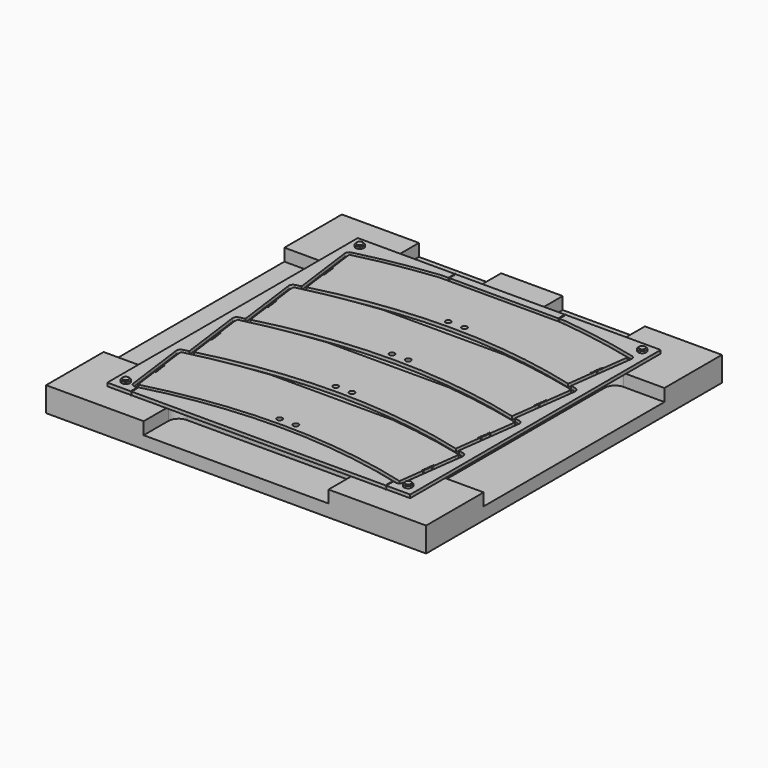
from build123d import *

# Parameters (mm, degrees)
F0_W     = 185
F0_H     = 180
F1_DEPTH = 12
F3_DEPTH = 6
F4_R     = 2.0005
F4_R_2   = 0.3015
F5_DEPTH = 1.6
F4_R_3   = 1.3005
F6_R     = 1.95
F7_DEPTH = 3
F8_SIZE  = 0.5


# Not quite as in the source:
# - ends of sketch curves that miss each other by under 0.0002 mm in the source are joined


with BuildPart() as f1:
    # F0 (on Top) → F1 (new body)
    with BuildSketch(Plane.XY):
        Rectangle(F0_W, F0_H)
    extrude(amount=F1_DEPTH)

    # F2 (on face) → F3 (cut)
    with BuildSketch(Plane.XY.offset(12)):
        with BuildLine():
            Line((117.5, -55), (117.5, 55))
            Line((117.5, 55), (72.5, 55))
            ThreePointArc((72.5, 55), (68.9644660941, 53.5355339059), (67.5, 50))
            Line((67.5, 50), (67.5, -50))
            ThreePointArc((67.5, -50), (68.9644660941, -53.5355339059), (72.5, -55))
            Line((72.5, -55), (117.5, -55))
        make_face()
        with BuildLine():
            ThreePointArc((45, -75), (43.5355339059, -71.4644660941), (40, -70))
            Line((40, -70), (-40, -70))
            ThreePointArc((-40, -70), (-43.5355339059, -71.4644660941), (-45, -75))
            Line((-45, -75), (-45, -110))
            Line((-45, -110), (45, -110))
            Line((45, -110), (45, -75))
        make_face()
        with BuildLine():
            Line((55, 77), (55, 108))
            Line((55, 108), (15, 108))
            Line((15, 108), (15, 77))
            ThreePointArc((15, 77), (16.4644660941, 73.4644660941), (20, 72))
            Line((20, 72), (50, 72))
            ThreePointArc((50, 72), (53.5355339059, 73.4644660941), (55, 77))
        make_face()
        with BuildLine():
            Line((-15, 108), (-55, 108))
            Line((-55, 108), (-55, 77))
            ThreePointArc((-55, 77), (-53.5355339059, 73.4644660941), (-50, 72))
            Line((-50, 72), (-20, 72))
            ThreePointArc((-20, 72), (-16.4644660941, 73.4644660941), (-15, 77))
            Line((-15, 77), (-15, 108))
        make_face()
        with BuildLine():
            ThreePointArc((-67.5, 50), (-68.9644660941, 53.5355339059), (-72.5, 55))
            Line((-72.5, 55), (-117.5, 55))
            Line((-117.5, 55), (-117.5, -55))
            Line((-117.5, -55), (-72.5, -55))
            ThreePointArc((-72.5, -55), (-68.9644660941, -53.5355339059), (-67.5, -50))
            Line((-67.5, -50), (-67.5, 50))
        make_face()
    extrude(amount=-F3_DEPTH, mode=Mode.SUBTRACT)

    # F6 (on face) → F7 (join)
    with BuildSketch(Plane.XY.offset(12)):
        with Locations((68.726, 71.2005)):
            Circle(F6_R)
        with Locations((-68.726, 71.2005)):
            Circle(F6_R)
        with Locations((68.726, -71.2005)):
            Circle(F6_R)
        with Locations((-68.726, -71.2005)):
            Circle(F6_R)
    extrude(amount=F7_DEPTH)

    # F8
    f8_edges = [f1.edges().sort_by_distance(p)[0] for p in [
        (-70.676, -71.2005, 15),
        (66.776, -71.2005, 15),
        (66.776, 71.2005, 15),
        (-70.676, 71.2005, 15),
    ]]
    chamfer(f8_edges, length=F8_SIZE)


with BuildPart() as f5:
    # F4 (on face) → F5 (new body)
    with BuildSketch(Plane.XY.offset(12)):
        with BuildLine():
            Line((-62.4545, -76.2005), (-61.8515, -76.2005))
            ThreePointArc((-61.8515, -76.2005), (-62.153, -75.899), (-62.4545, -76.2005))
        make_face()
        with BuildLine():
            ThreePointArc((-62.4545, -76.2005), (-62.153, -75.899), (-61.8515, -76.2005))
            Line((-61.8515, -76.2005), (61.5455, -76.2005))
            ThreePointArc((61.5455, -76.2005), (61.847, -75.899), (62.1485, -76.2005))
            Line((62.1485, -76.2005), (73.726, -76.2005))
            Line((73.726, -76.2005), (73.726, 76.2005))
            Line((73.726, 76.2005), (27.6285, 76.2005))
            ThreePointArc((27.6285, 76.2005), (27.327, 75.899), (27.0255, 76.2005))
            Line((27.0255, 76.2005), (-25.9215, 76.2005))
            ThreePointArc((-25.9215, 76.2005), (-26.223, 75.899), (-26.5245, 76.2005))
            Line((-26.5245, 76.2005), (-73.726, 76.2005))
            Line((-73.726, 76.2005), (-73.726, -76.2005))
            Line((-73.726, -76.2005), (-62.4545, -76.2005))
        make_face()
        with Locations((-68.726, -71.2005)):
            Circle(F4_R, mode=Mode.SUBTRACT)
        with Locations((-62.153, -75.2505)):
            Circle(F4_R_2, mode=Mode.SUBTRACT)
        with Locations((-62.153, -74.3005)):
            Circle(F4_R_2, mode=Mode.SUBTRACT)
        with Locations((-62.153, -73.3505)):
            Circle(F4_R_2, mode=Mode.SUBTRACT)
        with Locations((-62.153, -72.4005)):
            Circle(F4_R_2, mode=Mode.SUBTRACT)
        with Locations((61.847, -75.2505)):
            Circle(F4_R_2, mode=Mode.SUBTRACT)
        with Locations((61.847, -74.3005)):
            Circle(F4_R_2, mode=Mode.SUBTRACT)
        with Locations((61.847, -73.3505)):
            Circle(F4_R_2, mode=Mode.SUBTRACT)
        with Locations((61.847, -72.4005)):
            Circle(F4_R_2, mode=Mode.SUBTRACT)
        with Locations((68.726, -71.2005)):
            Circle(F4_R, mode=Mode.SUBTRACT)
        with BuildLine():
            Line((-65.62, -70.4485), (-67.2449358727, -58.1074915558))
            Line((-67.2449358727, -58.1074915558), (-69.709, -39.3935))
            ThreePointArc((-69.709, -39.3935), (-69.3772702277, -38.004016098), (-68.2030000316, -37.1904998711))
            Line((-68.2030000316, -37.1904998711), (-66.882, -36.8665))
            Line((-66.882, -36.8665), (-65.559, -36.5485))
            Line((-65.559, -36.5485), (-65.595, -36.3995))
            Line((-65.595, -36.3995), (-65.62, -36.2485))
            Line((-65.62, -36.2485), (-67.2450652985, -23.9065085973))
            Line((-67.2450652985, -23.9065085973), (-69.709, -5.1935))
            ThreePointArc((-69.709, -5.1935), (-69.3770638062, -3.8037858875), (-68.2029999873, -2.9895000517))
            Line((-68.2029999873, -2.9895000517), (-66.882, -2.6655))
            Line((-66.882, -2.6655), (-65.559, -2.3485))
            Line((-65.559, -2.3485), (-65.595, -2.1995))
            Line((-65.595, -2.1995), (-65.62, -2.0475))
            Line((-65.62, -2.0475), (-67.2449358727, 10.2935084442))
            Line((-67.2449358727, 10.2935084442), (-69.709, 29.0075))
            ThreePointArc((-69.709, 29.0075), (-69.3767664611, 30.3966415962), (-68.2030001005, 31.2105004081))
            Line((-68.2030001005, 31.2105004081), (-66.882, 31.5345))
            Line((-66.882, 31.5345), (-65.559, 31.8525))
            Line((-65.559, 31.8525), (-65.595, 32.0015))
            Line((-65.595, 32.0015), (-65.62, 32.1525))
            Line((-65.62, 32.1525), (-67.2449358727, 44.4935084442))
            Line((-67.2449358727, 44.4935084442), (-69.709, 63.2075))
            ThreePointArc((-69.709, 63.2075), (-69.3772702277, 64.596983902), (-68.2030000316, 65.4105001289))
            ThreePointArc((-68.2030000316, 65.4105001289), (-49.0501556944, 69.4631942467), (-29.6639999694, 72.1894997101))
            Line((-29.6639999694, 72.1894997101), (-29.557, 72.1985))
            Line((-29.557, 72.1985), (-29.449, 72.2015))
            Line((-29.449, 72.2015), (-26.4494533888, 72.201449472))
            ThreePointArc((-26.4494533888, 72.201449472), (-26.3293638879, 72.6826151775), (-25.9215, 72.4005))
            ThreePointArc((-25.9215, 72.4005), (-25.9408866143, 72.2941313599), (-25.9965533175, 72.2014418428))
            Line((-25.9965533175, 72.2014418428), (27.1013427235, 72.2005473967))
            ThreePointArc((27.1013427235, 72.2005473967), (27.2200734338, 72.6824023934), (27.6285, 72.4005))
            ThreePointArc((27.6285, 72.4005), (27.6089005922, 72.2935686851), (27.5526505399, 72.2005397943))
            Line((27.5526505399, 72.2005397943), (29.915, 72.2005))
            Line((29.915, 72.2005), (29.924, 72.2005))
            Line((29.924, 72.2005), (30.031, 72.1975))
            Line((30.031, 72.1975), (30.137, 72.1885))
            ThreePointArc((30.137, 72.1885), (49.2837916508, 69.5048541336), (68.2040000196, 65.5265000796))
            ThreePointArc((68.2040000196, 65.5265000796), (69.3770080847, 64.7122741999), (69.7089998684, 63.3235000172))
            Line((69.7089998684, 63.3235000172), (68.0082998947, 50.4077430393))
            Line((68.0082998947, 50.4077430393), (67.2342399079, 44.5292400436))
            Line((67.2342399079, 44.5292400436), (65.619, 32.2625))
            Line((65.619, 32.2625), (65.594, 32.1115))
            Line((65.594, 32.1115), (65.557, 31.9635))
            Line((65.557, 31.9635), (66.881, 31.6475))
            Line((66.881, 31.6475), (68.204, 31.3255))
            ThreePointArc((68.204, 31.3255), (69.3774420415, 30.5115704613), (69.7090000669, 29.1224999912))
            Line((69.7090000669, 29.1224999912), (68.0089998907, 16.212059072))
            Line((68.0089998907, 16.212059072), (67.2342480853, 10.3283021459))
            Line((67.2342480853, 10.3283021459), (65.619, -1.9385))
            Line((65.619, -1.9385), (65.594, -2.0885))
            Line((65.594, -2.0885), (65.557, -2.2365))
            Line((65.557, -2.2365), (66.881, -2.5525))
            Line((66.881, -2.5525), (68.204, -2.8745))
            ThreePointArc((68.204, -2.8745), (69.3770080847, -3.6887258001), (69.7089998684, -5.0774999828))
            Line((69.7089998684, -5.0774999828), (68.0089998907, -17.987940928))
            Line((68.0089998907, -17.987940928), (67.2342399079, -23.8717599564))
            Line((67.2342399079, -23.8717599564), (65.619, -36.1385))
            Line((65.619, -36.1385), (65.594, -36.2895))
            Line((65.594, -36.2895), (65.557, -36.4365))
            Line((65.557, -36.4365), (66.881, -36.7525))
            Line((66.881, -36.7525), (68.204, -37.0745))
            ThreePointArc((68.204, -37.0745), (69.3770080847, -37.8887258001), (69.7089998684, -39.2774999828))
            Line((69.7089998684, -39.2774999828), (69.709, -39.2785))
            Line((69.709, -39.2785), (68.0098089454, -52.1827966615))
            Line((68.0098089454, -52.1827966615), (67.233899191, -58.0753474888))
            Line((67.233899191, -58.0753474888), (65.619, -70.3395))
            ThreePointArc((65.619, -70.3395), (64.749919219, -71.7392145375), (63.1250000615, -72.0114997676))
            ThreePointArc((63.1250000615, -72.0114997676), (-0.0064015619, -63.8958856781), (-63.1220000549, -72.1334997925))
            Line((-63.1220000549, -72.1334997925), (-63.124, -72.1335))
            ThreePointArc((-63.124, -72.1335), (-64.7548109583, -71.858060865), (-65.62, -70.4485))
        make_face(mode=Mode.SUBTRACT)
        with Locations((-68.726, 71.2005)):
            Circle(F4_R, mode=Mode.SUBTRACT)
        with Locations((-26.223, 73.3505)):
            Circle(F4_R_2, mode=Mode.SUBTRACT)
        with Locations((-26.223, 74.3005)):
            Circle(F4_R_2, mode=Mode.SUBTRACT)
        with Locations((-26.223, 75.2505)):
            Circle(F4_R_2, mode=Mode.SUBTRACT)
        with Locations((27.327, 73.3505)):
            Circle(F4_R_2, mode=Mode.SUBTRACT)
        with Locations((27.327, 74.3005)):
            Circle(F4_R_2, mode=Mode.SUBTRACT)
        with Locations((27.327, 75.2505)):
            Circle(F4_R_2, mode=Mode.SUBTRACT)
        with Locations((68.726, 71.2005)):
            Circle(F4_R, mode=Mode.SUBTRACT)
        with BuildLine():
            ThreePointArc((-62.4545, -76.2005), (-62.153, -76.502), (-61.8515, -76.2005))
            Line((-61.8515, -76.2005), (-62.4545, -76.2005))
        make_face()
        with BuildLine():
            Line((62.1485, -76.2005), (61.5455, -76.2005))
            ThreePointArc((61.5455, -76.2005), (61.847, -76.502), (62.1485, -76.2005))
        make_face()
        with BuildLine():
            ThreePointArc((62.1485, -76.2005), (61.847, -75.899), (61.5455, -76.2005))
            Line((61.5455, -76.2005), (62.1485, -76.2005))
        make_face()
        with BuildLine():
            Line((-25.9215, 76.2005), (-26.5245, 76.2005))
            ThreePointArc((-26.5245, 76.2005), (-26.223, 75.899), (-25.9215, 76.2005))
        make_face()
        with BuildLine():
            ThreePointArc((-25.9215, 76.2005), (-26.223, 76.502), (-26.5245, 76.2005))
            Line((-26.5245, 76.2005), (-25.9215, 76.2005))
        make_face()
        with BuildLine():
            Line((27.0255, 76.2005), (27.6285, 76.2005))
            ThreePointArc((27.6285, 76.2005), (27.327, 76.502), (27.0255, 76.2005))
        make_face()
        with BuildLine():
            ThreePointArc((27.0255, 76.2005), (27.327, 75.899), (27.6285, 76.2005))
            Line((27.6285, 76.2005), (27.0255, 76.2005))
        make_face()
    extrude(amount=F5_DEPTH)


with BuildPart() as f5b:
    # F4 (on face) → F5, piece 2 (new body)
    with BuildSketch(Plane.XY.offset(12)):
        with BuildLine():
            Line((-65.2784456317, 44.8756615856), (-65.2664345686, 44.784424493))
            Line((-65.2664345686, 44.784424493), (-63.636, 32.3995))
            ThreePointArc((-63.636, 32.3995), (-0.007966778, 40.7044773709), (63.6359999804, 32.5224999254))
            Line((63.6359999804, 32.5224999254), (63.637, 32.5225))
            Line((63.637, 32.5225), (65.247008228, 44.7524989168))
            Line((65.247008228, 44.7524989168), (65.2625989091, 44.8709293753))
            ThreePointArc((65.2625989091, 44.8709293753), (64.669481786, 44.9740121639), (65.2705, 44.9395))
            ThreePointArc((65.2705, 44.9395), (65.2704605754, 44.934624399), (65.2703423119, 44.9297500732))
            Line((65.2703423119, 44.9297500732), (65.3866191433, 45.8130160697))
            ThreePointArc((65.3866191433, 45.8130160697), (64.793476694, 45.9159679438), (65.3945, 45.8815))
            ThreePointArc((65.3945, 45.8815), (65.3944598523, 45.8765798927), (65.3943394199, 45.8716610957))
            Line((65.3943394199, 45.8716610957), (65.5106394125, 46.7551030307))
            ThreePointArc((65.5106394125, 46.7551030307), (64.9174715933, 46.8579235902), (65.5185, 46.8235))
            ThreePointArc((65.5185, 46.8235), (65.5184591204, 46.8185352527), (65.5183364928, 46.8135718517))
            Line((65.5183364928, 46.8135718517), (65.6346597172, 47.6971902605))
            ThreePointArc((65.6346597172, 47.6971902605), (65.0414664837, 47.7998791017), (65.6425, 47.7655))
            ThreePointArc((65.6425, 47.7655), (65.6424583797, 47.7604904779), (65.6423335303, 47.7554823389))
            Line((65.6423335303, 47.7554823389), (65.7586800576, 48.6392777617))
            ThreePointArc((65.7586800576, 48.6392777617), (65.1654613653, 48.7418344772), (65.7665, 48.7075))
            ThreePointArc((65.7665, 48.7075), (65.76645763, 48.7024455671), (65.7663305321, 48.6973925547))
            Line((65.7663305321, 48.6973925547), (65.882700434, 49.5813655368))
            ThreePointArc((65.882700434, 49.5813655368), (65.2894562379, 49.6837897153), (65.8905, 49.6495))
            ThreePointArc((65.8905, 49.6495), (65.8904568714, 49.6444005189), (65.8903274978, 49.6393024967))
            Line((65.8903274978, 49.6393024967), (66.0067208468, 50.5234535882))
            ThreePointArc((66.0067208468, 50.5234535882), (65.4134511014, 50.6257448149), (66.0145, 50.5915))
            ThreePointArc((66.0145, 50.5915), (66.0144561036, 50.5863553321), (66.0143244271, 50.5812121623))
            Line((66.0143244271, 50.5812121623), (66.0300275006, 50.7004963797))
            Line((66.0300275006, 50.7004963797), (67.726, 63.5835))
            ThreePointArc((67.726, 63.5835), (48.9375198691, 67.5344075087), (29.9239999395, 70.1994994278))
            Line((29.9239999395, 70.1994994278), (-29.449, 70.2005))
            ThreePointArc((-29.449, 70.2005), (-48.7034920703, 67.4934131145), (-67.7259999773, 63.4674999085))
            Line((-67.7259999773, 63.4674999085), (-66.0410699573, 50.668623089))
            Line((-66.0410699573, 50.668623089), (-66.0291576494, 50.5781361497))
            ThreePointArc((-66.0291576494, 50.5781361497), (-65.7351839648, 50.8939144002), (-65.4265, 50.5925))
            ThreePointArc((-65.4265, 50.5925), (-65.6957817363, 50.2927263629), (-66.0226143183, 50.5284324306))
            Line((-66.0226143183, 50.5284324306), (-65.905163967, 49.6362692241))
            ThreePointArc((-65.905163967, 49.6362692241), (-65.6111173714, 49.95191598), (-65.3025, 49.6505))
            ThreePointArc((-65.3025, 49.6505), (-65.5717155063, 49.3507334884), (-65.8985859799, 49.5863022551))
            Line((-65.8985859799, 49.5863022551), (-65.7811701931, 48.6944016039))
            ThreePointArc((-65.7811701931, 48.6944016039), (-65.4870511266, 49.009917537), (-65.1785, 48.7085))
            ThreePointArc((-65.1785, 48.7085), (-65.447649625, 48.4087405911), (-65.7745577329, 48.6441727743))
            Line((-65.7745577329, 48.6441727743), (-65.6571763292, 47.7525332999))
            ThreePointArc((-65.6571763292, 47.7525332999), (-65.362985225, 48.0679190714), (-65.0545, 47.7665))
            ThreePointArc((-65.0545, 47.7665), (-65.323584087, 47.4667476713), (-65.650529576, 47.7020439773))
            Line((-65.650529576, 47.7020439773), (-65.5331823767, 46.8106643225))
            ThreePointArc((-65.5331823767, 46.8106643225), (-65.2389196614, 47.1259205837), (-64.9305, 46.8245))
            ThreePointArc((-64.9305, 46.8245), (-65.1995188868, 46.5247547293), (-65.5265015077, 46.7599158537))
            Line((-65.5265015077, 46.7599158537), (-65.4091883369, 45.868794682))
            ThreePointArc((-65.4091883369, 45.868794682), (-65.1148544306, 46.1839220741), (-64.8065, 45.8825))
            ThreePointArc((-64.8065, 45.8825), (-65.0754540195, 45.5827617656), (-65.4024735267, 45.8177883931))
            Line((-65.4024735267, 45.8177883931), (-65.2851942111, 44.9269243885))
            ThreePointArc((-65.2851942111, 44.9269243885), (-64.9907895275, 45.2419235431), (-64.6825, 44.9405))
            ThreePointArc((-64.6825, 44.9405), (-64.9513894799, 44.6407687804), (-65.2784456317, 44.8756615856))
        make_face()
        with Locations((-3.938, 44.0025)):
            Circle(F4_R_3, mode=Mode.SUBTRACT)
        with Locations((3.962, 44.0025)):
            Circle(F4_R_3, mode=Mode.SUBTRACT)
    extrude(amount=F5_DEPTH)


with BuildPart() as f5c:
    # F4 (on face) → F5, piece 3 (new body)
    with BuildSketch(Plane.XY.offset(12)):
        with BuildLine():
            ThreePointArc((-29.448999994, 36.0004999433), (-48.5888395368, 33.3135563554), (-67.5, 29.323426846))
            Line((-67.5, 29.323426846), (-67.5, 27.5507841076))
            Line((-67.5, 27.5507841076), (-66.0410699573, 16.468623089))
            Line((-66.0410699573, 16.468623089), (-66.0291576494, 16.3781361497))
            ThreePointArc((-66.0291576494, 16.3781361497), (-65.7351839648, 16.6939144002), (-65.4265, 16.3925))
            ThreePointArc((-65.4265, 16.3925), (-65.6957817363, 16.0927263629), (-66.0226143183, 16.3284324306))
            Line((-66.0226143183, 16.3284324306), (-65.905163967, 15.4362692241))
            ThreePointArc((-65.905163967, 15.4362692241), (-65.6111173714, 15.75191598), (-65.3025, 15.4505))
            ThreePointArc((-65.3025, 15.4505), (-65.5717155063, 15.1507334884), (-65.8985859799, 15.3863022551))
            Line((-65.8985859799, 15.3863022551), (-65.7811701931, 14.4944016039))
            ThreePointArc((-65.7811701931, 14.4944016039), (-65.4870511266, 14.809917537), (-65.1785, 14.5085))
            ThreePointArc((-65.1785, 14.5085), (-65.447649625, 14.2087405911), (-65.7745577329, 14.4441727743))
            Line((-65.7745577329, 14.4441727743), (-65.6571763292, 13.5525332999))
            ThreePointArc((-65.6571763292, 13.5525332999), (-65.362985225, 13.8679190714), (-65.0545, 13.5665))
            ThreePointArc((-65.0545, 13.5665), (-65.323584087, 13.2667476713), (-65.650529576, 13.5020439773))
            Line((-65.650529576, 13.5020439773), (-65.5331823767, 12.6106643225))
            ThreePointArc((-65.5331823767, 12.6106643225), (-65.2389196614, 12.9259205837), (-64.9305, 12.6245))
            ThreePointArc((-64.9305, 12.6245), (-65.1995188868, 12.3247547293), (-65.5265015077, 12.5599158537))
            Line((-65.5265015077, 12.5599158537), (-65.4091883369, 11.668794682))
            ThreePointArc((-65.4091883369, 11.668794682), (-65.1148544306, 11.9839220741), (-64.8065, 11.6825))
            ThreePointArc((-64.8065, 11.6825), (-65.0754540195, 11.3827617656), (-65.4024735267, 11.6177883931))
            Line((-65.4024735267, 11.6177883931), (-65.2851942111, 10.7269243885))
            ThreePointArc((-65.2851942111, 10.7269243885), (-64.9907895275, 11.0419235431), (-64.6825, 10.7405))
            ThreePointArc((-64.6825, 10.7405), (-64.9513894799, 10.4407687804), (-65.2784456317, 10.6756615856))
            Line((-65.2784456317, 10.6756615856), (-65.2664345686, 10.584424493))
            Line((-65.2664345686, 10.584424493), (-63.636, -1.8005))
            ThreePointArc((-63.636, -1.8005), (-0.007966778, 6.5044773709), (63.6359999804, -1.6775000746))
            Line((63.6359999804, -1.6775000746), (63.637, -1.6775))
            Line((63.637, -1.6775), (65.2470082281, 10.5524989175))
            Line((65.2470082281, 10.5524989175), (65.2625989091, 10.6709293753))
            ThreePointArc((65.2625989091, 10.6709293753), (64.669481786, 10.7740121639), (65.2705, 10.7395))
            ThreePointArc((65.2705, 10.7395), (65.2704605754, 10.734624399), (65.2703423119, 10.7297500732))
            Line((65.2703423119, 10.7297500732), (65.3866191433, 11.6130160697))
            ThreePointArc((65.3866191433, 11.6130160697), (64.793476694, 11.7159679438), (65.3945, 11.6815))
            ThreePointArc((65.3945, 11.6815), (65.3944598523, 11.6765798927), (65.3943394199, 11.6716610957))
            Line((65.3943394199, 11.6716610957), (65.5106394125, 12.5551030307))
            ThreePointArc((65.5106394125, 12.5551030307), (64.9174715933, 12.6579235902), (65.5185, 12.6235))
            ThreePointArc((65.5185, 12.6235), (65.5184591204, 12.6185352527), (65.5183364928, 12.6135718517))
            Line((65.5183364928, 12.6135718517), (65.6346597172, 13.4971902605))
            ThreePointArc((65.6346597172, 13.4971902605), (65.0414664837, 13.5998791017), (65.6425, 13.5655))
            ThreePointArc((65.6425, 13.5655), (65.6424583797, 13.5604904779), (65.6423335303, 13.5554823389))
            Line((65.6423335303, 13.5554823389), (65.7586800576, 14.4392777617))
            ThreePointArc((65.7586800576, 14.4392777617), (65.1654613653, 14.5418344772), (65.7665, 14.5075))
            ThreePointArc((65.7665, 14.5075), (65.76645763, 14.5024455671), (65.7663305321, 14.4973925547))
            Line((65.7663305321, 14.4973925547), (65.882700434, 15.3813655368))
            ThreePointArc((65.882700434, 15.3813655368), (65.2894562379, 15.4837897153), (65.8905, 15.4495))
            ThreePointArc((65.8905, 15.4495), (65.8904568714, 15.4444005189), (65.8903274978, 15.4393024967))
            Line((65.8903274978, 15.4393024967), (66.0067208468, 16.3234535882))
            ThreePointArc((66.0067208468, 16.3234535882), (65.4134511014, 16.4257448149), (66.0145, 16.3915))
            ThreePointArc((66.0145, 16.3915), (66.0144561036, 16.3863553321), (66.0143244271, 16.3812121623))
            Line((66.0143244271, 16.3812121623), (66.0300275006, 16.5004963797))
            Line((66.0300275006, 16.5004963797), (67.5, 27.6667511617))
            Line((67.5, 27.6667511617), (67.5, 29.4390097901))
            ThreePointArc((67.5, 29.4390097901), (48.8228992609, 33.3544437485), (29.9239999395, 35.9994994278))
            Line((29.9239999395, 35.9994994278), (-29.448999994, 36.0004999433))
        make_face()
        with Locations((-3.938, 9.8025)):
            Circle(F4_R_3, mode=Mode.SUBTRACT)
        with Locations((3.962, 9.8025)):
            Circle(F4_R_3, mode=Mode.SUBTRACT)
    extrude(amount=F5_DEPTH)


with BuildPart() as f5d:
    # F4 (on face) → F5, piece 4 (new body)
    with BuildSketch(Plane.XY.offset(12)):
        with BuildLine():
            Line((-65.2784456317, -23.5243384144), (-65.2664345686, -23.615575507))
            Line((-65.2664345686, -23.615575507), (-63.636, -36.0005))
            ThreePointArc((-63.636, -36.0005), (-0.007966778, -27.6955226291), (63.6359999804, -35.8775000746))
            Line((63.6359999804, -35.8775000746), (63.637, -35.8775))
            Line((63.637, -35.8775), (65.2625989091, -23.5290706247))
            ThreePointArc((65.2625989091, -23.5290706247), (64.669481786, -23.4259878361), (65.2705, -23.4605))
            ThreePointArc((65.2705, -23.4605), (65.2704605754, -23.465375601), (65.2703423119, -23.4702499268))
            Line((65.2703423119, -23.4702499268), (65.3866191433, -22.5869839303))
            ThreePointArc((65.3866191433, -22.5869839303), (64.793476694, -22.4840320562), (65.3945, -22.5185))
            ThreePointArc((65.3945, -22.5185), (65.3944598523, -22.5234201073), (65.3943394199, -22.5283389043))
            Line((65.3943394199, -22.5283389043), (65.5106394125, -21.6448969693))
            ThreePointArc((65.5106394125, -21.6448969693), (64.9174715933, -21.5420764098), (65.5185, -21.5765))
            ThreePointArc((65.5185, -21.5765), (65.5184591204, -21.5814647473), (65.5183364928, -21.5864281483))
            Line((65.5183364928, -21.5864281483), (65.6346597172, -20.7028097395))
            ThreePointArc((65.6346597172, -20.7028097395), (65.0414664837, -20.6001208983), (65.6425, -20.6345))
            ThreePointArc((65.6425, -20.6345), (65.6424583797, -20.6395095221), (65.6423335303, -20.6445176611))
            Line((65.6423335303, -20.6445176611), (65.7586800576, -19.7607222383))
            ThreePointArc((65.7586800576, -19.7607222383), (65.1654613653, -19.6581655228), (65.7665, -19.6925))
            ThreePointArc((65.7665, -19.6925), (65.76645763, -19.6975544329), (65.7663305321, -19.7026074453))
            Line((65.7663305321, -19.7026074453), (65.882700434, -18.8186344632))
            ThreePointArc((65.882700434, -18.8186344632), (65.2894562379, -18.7162102847), (65.8905, -18.7505))
            ThreePointArc((65.8905, -18.7505), (65.8904568714, -18.7555994811), (65.8903274978, -18.7606975033))
            Line((65.8903274978, -18.7606975033), (66.0067208468, -17.8765464118))
            ThreePointArc((66.0067208468, -17.8765464118), (65.4134511014, -17.7742551851), (66.0145, -17.8085))
            ThreePointArc((66.0145, -17.8085), (66.0144561036, -17.8136446679), (66.0143244271, -17.8187878377))
            Line((66.0143244271, -17.8187878377), (66.0300275006, -17.6995036203))
            Line((66.0300275006, -17.6995036203), (67.5, -6.5332488383))
            Line((67.5, -6.5332488383), (67.5, -4.7609902099))
            ThreePointArc((67.5, -4.7609902099), (48.8228992609, -0.8455562515), (29.9239999395, 1.7994994278))
            Line((29.9239999395, 1.7994994278), (-29.449, 1.8005))
            ThreePointArc((-29.449, 1.8005), (-48.5888395368, -0.8864436446), (-67.5, -4.876573154))
            Line((-67.5, -4.876573154), (-67.5, -6.6492158924))
            Line((-67.5, -6.6492158924), (-66.0414363548, -17.7285937236))
            Line((-66.0414363548, -17.7285937236), (-66.0291576494, -17.8218638503))
            ThreePointArc((-66.0291576494, -17.8218638503), (-65.7351839648, -17.5060855998), (-65.4265, -17.8075))
            ThreePointArc((-65.4265, -17.8075), (-65.6957817363, -18.1072736371), (-66.0226143183, -17.8715675694))
            Line((-66.0226143183, -17.8715675694), (-65.905163967, -18.7637307759))
            ThreePointArc((-65.905163967, -18.7637307759), (-65.6111173714, -18.44808402), (-65.3025, -18.7495))
            ThreePointArc((-65.3025, -18.7495), (-65.5717155063, -19.0492665116), (-65.8985859799, -18.8136977449))
            Line((-65.8985859799, -18.8136977449), (-65.7811701931, -19.7055983961))
            ThreePointArc((-65.7811701931, -19.7055983961), (-65.4870511266, -19.390082463), (-65.1785, -19.6915))
            ThreePointArc((-65.1785, -19.6915), (-65.447649625, -19.9912594089), (-65.7745577329, -19.7558272257))
            Line((-65.7745577329, -19.7558272257), (-65.6571763292, -20.6474667001))
            ThreePointArc((-65.6571763292, -20.6474667001), (-65.362985225, -20.3320809286), (-65.0545, -20.6335))
            ThreePointArc((-65.0545, -20.6335), (-65.323584087, -20.9332523287), (-65.650529576, -20.6979560227))
            Line((-65.650529576, -20.6979560227), (-65.5331823767, -21.5893356775))
            ThreePointArc((-65.5331823767, -21.5893356775), (-65.2389196614, -21.2740794163), (-64.9305, -21.5755))
            ThreePointArc((-64.9305, -21.5755), (-65.1995188868, -21.8752452707), (-65.5265015077, -21.6400841463))
            Line((-65.5265015077, -21.6400841463), (-65.4091883369, -22.531205318))
            ThreePointArc((-65.4091883369, -22.531205318), (-65.1148544306, -22.2160779259), (-64.8065, -22.5175))
            ThreePointArc((-64.8065, -22.5175), (-65.0754540195, -22.8172382344), (-65.4024735267, -22.5822116069))
            Line((-65.4024735267, -22.5822116069), (-65.2851942111, -23.4730756115))
            ThreePointArc((-65.2851942111, -23.4730756115), (-64.9907895275, -23.1580764569), (-64.6825, -23.4595))
            ThreePointArc((-64.6825, -23.4595), (-64.9513894799, -23.7592312196), (-65.2784456317, -23.5243384144))
        make_face()
        with Locations((-3.938, -24.3975)):
            Circle(F4_R_3, mode=Mode.SUBTRACT)
        with Locations((3.962, -24.3975)):
            Circle(F4_R_3, mode=Mode.SUBTRACT)
    extrude(amount=F5_DEPTH)


with BuildPart() as f5e:
    # F4 (on face) → F5, piece 5 (new body)
    with BuildSketch(Plane.XY.offset(12)):
        with BuildLine():
            ThreePointArc((-65.7811701931, -53.9055983961), (-65.4870511266, -53.590082463), (-65.1785, -53.8915))
            ThreePointArc((-65.1785, -53.8915), (-65.447649625, -54.1912594089), (-65.7745577329, -53.9558272257))
            Line((-65.7745577329, -53.9558272257), (-65.6571763292, -54.8474667001))
            ThreePointArc((-65.6571763292, -54.8474667001), (-65.362985225, -54.5320809286), (-65.0545, -54.8335))
            ThreePointArc((-65.0545, -54.8335), (-65.323584087, -55.1332523287), (-65.650529576, -54.8979560227))
            Line((-65.650529576, -54.8979560227), (-65.5331823767, -55.7893356775))
            ThreePointArc((-65.5331823767, -55.7893356775), (-65.2389196614, -55.4740794163), (-64.9305, -55.7755))
            ThreePointArc((-64.9305, -55.7755), (-65.1995188868, -56.0752452707), (-65.5265015077, -55.8400841463))
            Line((-65.5265015077, -55.8400841463), (-65.4091883369, -56.731205318))
            ThreePointArc((-65.4091883369, -56.731205318), (-65.1148544306, -56.4160779259), (-64.8065, -56.7175))
            ThreePointArc((-64.8065, -56.7175), (-65.0754540195, -57.0172382344), (-65.4024735267, -56.7822116069))
            Line((-65.4024735267, -56.7822116069), (-65.2851942111, -57.6730756115))
            ThreePointArc((-65.2851942111, -57.6730756115), (-64.9907895275, -57.3580764569), (-64.6825, -57.6595))
            ThreePointArc((-64.6825, -57.6595), (-64.9513894799, -57.9592312196), (-65.2784456317, -57.7243384144))
            Line((-65.2784456317, -57.7243384144), (-65.2657199583, -57.8210037493))
            Line((-65.2657199583, -57.8210037493), (-63.636, -70.2005))
            ThreePointArc((-63.636, -70.2005), (-0.007966778, -61.8955226291), (63.6359999804, -70.0775000746))
            Line((63.6359999804, -70.0775000746), (63.637, -70.0775))
            Line((63.637, -70.0775), (65.2625989091, -57.7290706247))
            ThreePointArc((65.2625989091, -57.7290706247), (64.669481786, -57.6259878361), (65.2705, -57.6605))
            ThreePointArc((65.2705, -57.6605), (65.2704605754, -57.665375601), (65.2703423119, -57.6702499268))
            Line((65.2703423119, -57.6702499268), (65.3866191433, -56.7869839303))
            ThreePointArc((65.3866191433, -56.7869839303), (64.793476694, -56.6840320562), (65.3945, -56.7185))
            ThreePointArc((65.3945, -56.7185), (65.3944598523, -56.7234201073), (65.3943394199, -56.7283389043))
            Line((65.3943394199, -56.7283389043), (65.5106394125, -55.8448969693))
            ThreePointArc((65.5106394125, -55.8448969693), (64.9174715933, -55.7420764098), (65.5185, -55.7765))
            ThreePointArc((65.5185, -55.7765), (65.5184591204, -55.7814647473), (65.5183364928, -55.7864281483))
            Line((65.5183364928, -55.7864281483), (65.6346597172, -54.9028097395))
            ThreePointArc((65.6346597172, -54.9028097395), (65.0414664837, -54.8001208983), (65.6425, -54.8345))
            ThreePointArc((65.6425, -54.8345), (65.6424583797, -54.8395095221), (65.6423335303, -54.8445176611))
            Line((65.6423335303, -54.8445176611), (65.7586800576, -53.9607222383))
            ThreePointArc((65.7586800576, -53.9607222383), (65.1654613653, -53.8581655228), (65.7665, -53.8925))
            ThreePointArc((65.7665, -53.8925), (65.76645763, -53.8975544329), (65.7663305321, -53.9026074453))
            Line((65.7663305321, -53.9026074453), (65.882700434, -53.0186344632))
            ThreePointArc((65.882700434, -53.0186344632), (65.2894562379, -52.9162102847), (65.8905, -52.9505))
            ThreePointArc((65.8905, -52.9505), (65.8904568714, -52.9555994811), (65.8903274978, -52.9606975033))
            Line((65.8903274978, -52.9606975033), (66.0067208468, -52.0765464118))
            ThreePointArc((66.0067208468, -52.0765464118), (65.4134511014, -51.9742551851), (66.0145, -52.0085))
            ThreePointArc((66.0145, -52.0085), (66.0144561036, -52.0136446679), (66.0143244271, -52.0187878377))
            Line((66.0143244271, -52.0187878377), (66.0300275006, -51.8995036203))
            Line((66.0300275006, -51.8995036203), (67.5, -40.7332488383))
            Line((67.5, -40.7332488383), (67.5, -38.9609902099))
            ThreePointArc((67.5, -38.9609902099), (48.8228992609, -35.0455562515), (29.9239999395, -32.4005005722))
            Line((29.9239999395, -32.4005005722), (-29.449, -32.3995))
            ThreePointArc((-29.449, -32.3995), (-48.5888395368, -35.0864436446), (-67.5, -39.076573154))
            Line((-67.5, -39.076573154), (-67.5, -40.8492158924))
            Line((-67.5, -40.8492158924), (-66.0414363548, -51.9285937236))
            Line((-66.0414363548, -51.9285937236), (-66.0291576494, -52.0218638503))
            ThreePointArc((-66.0291576494, -52.0218638503), (-65.7351839648, -51.7060855998), (-65.4265, -52.0075))
            ThreePointArc((-65.4265, -52.0075), (-65.6957817363, -52.3072736371), (-66.0226143183, -52.0715675694))
            Line((-66.0226143183, -52.0715675694), (-65.905163967, -52.9637307759))
            ThreePointArc((-65.905163967, -52.9637307759), (-65.6111173714, -52.64808402), (-65.3025, -52.9495))
            ThreePointArc((-65.3025, -52.9495), (-65.5717155063, -53.2492665116), (-65.8985859799, -53.0136977449))
            Line((-65.8985859799, -53.0136977449), (-65.7811701931, -53.9055983961))
        make_face()
        with Locations((-3.938, -58.5975)):
            Circle(F4_R_3, mode=Mode.SUBTRACT)
        with Locations((3.962, -58.5975)):
            Circle(F4_R_3, mode=Mode.SUBTRACT)
    extrude(amount=F5_DEPTH)


solid = Compound([f1.part, f5.part, f5b.part, f5c.part, f5d.part, f5e.part])
